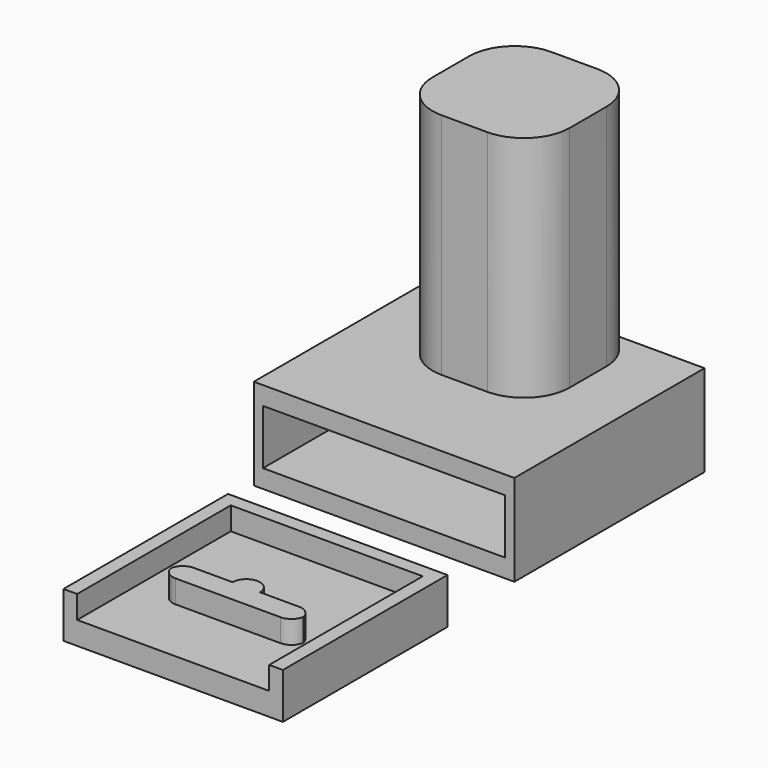
from build123d import *

# Parameters (mm, degrees)
F0_W        = 42
F0_H        = 39
F0_H_2      = 3
F1_DEPTH    = 5
F2_DEPTH    = 5
F3_T1_DEPTH = 12.5
F4_DEPTH    = 20
F0_W_2      = 53
F0_H_3      = 50
F5_DEPTH    = 4
F6_W        = 53
F6_H        = 4
F7_DEPTH    = 50
F8_W        = 30
F8_H        = 30
F9_DEPTH    = 50
F10_R       = 10


# Not quite as in the source:
# - a fillet or chamfer that OpenCascade refuses, or shapes differently, is made with other operations: its cross-section is extruded or revolved along the edge and cut away or added


with BuildPart() as f1:
    # F0 (on Top) → F1 (new body)
    with BuildSketch(Plane.XY):
        Rectangle(F0_W, F0_H)
        Polygon((-14.5, -7.5), (-14.5, -2.5), (-3, -2.5), (-3, 0.5), (3, 0.5), (3, -2.5), (14.5, -2.5), (14.5, -7.5), (3, -7.5), (-3, -7.5), align=None, mode=Mode.SUBTRACT)
        Polygon((-21, 19.5), (21, 19.5), (21, -19.5), (21, -22.5), (24, -22.5), (24, 22.5), (-24, 22.5), (-24, -22.5), (-21, -22.5), (-21, -19.5), align=None)
        with Locations((0, -21)):
            Rectangle(F0_W, F0_H_2)
        Polygon((-3, -2.5), (-14.5, -2.5), (-14.5, -7.5), (-3, -7.5), (3, -7.5), (14.5, -7.5), (14.5, -2.5), (3, -2.5), (3, 0.5), (-3, 0.5), align=None)
    extrude(amount=-F1_DEPTH)

    # F0 (on Top) → F2 (join)
    with BuildSketch(Plane.XY):
        Polygon((-3, -2.5), (-14.5, -2.5), (-14.5, -7.5), (-3, -7.5), (3, -7.5), (14.5, -7.5), (14.5, -2.5), (3, -2.5), (3, 0.5), (-3, 0.5), align=None)
        Polygon((-21, 19.5), (21, 19.5), (21, -19.5), (21, -22.5), (24, -22.5), (24, 22.5), (-24, 22.5), (-24, -22.5), (-21, -22.5), (-21, -19.5), align=None)
    extrude(amount=F2_DEPTH)

    # F3: fillet of radius 3 on 6 edges, made by hand

    # F3_s2 → F3_t1 (cut)
    with BuildSketch(Plane.XY):
        with BuildLine():
            ThreePointArc((-3, -2.5), (-2.1213203436, -0.3786796564), (0, 0.5))
            Line((0, 0.5), (-3, 0.5))
            Line((-3, 0.5), (-3, -2.5))
        make_face()
        with BuildLine():
            ThreePointArc((0, 0.5), (2.1213203436, -0.3786796564), (3, -2.5))
            Line((3, -2.5), (3, 0.5))
            Line((3, 0.5), (0, 0.5))
        make_face()
        with BuildLine():
            ThreePointArc((-14.5, -5.5), (-13.6213203436, -3.3786796564), (-11.5, -2.5))
            Line((-11.5, -2.5), (-14.5, -2.5))
            Line((-14.5, -2.5), (-14.5, -5.5))
        make_face()
        with BuildLine():
            ThreePointArc((-11.5, -7.5), (-13.6213203436, -6.6213203436), (-14.5, -4.5))
            Line((-14.5, -4.5), (-14.5, -7.5))
            Line((-14.5, -7.5), (-11.5, -7.5))
        make_face()
        with BuildLine():
            ThreePointArc((11.5, -2.5), (13.6213203436, -3.3786796564), (14.5, -5.5))
            Line((14.5, -5.5), (14.5, -2.5))
            Line((14.5, -2.5), (11.5, -2.5))
        make_face()
        with BuildLine():
            ThreePointArc((14.5, -4.5), (13.6213203436, -6.6213203436), (11.5, -7.5))
            Line((11.5, -7.5), (14.5, -7.5))
            Line((14.5, -7.5), (14.5, -4.5))
        make_face()
    extrude(amount=F3_T1_DEPTH, mode=Mode.SUBTRACT)


with BuildPart() as f4:
    # F0 (on Top) → F4 (new body)
    with BuildSketch(Plane.XY):
        Polygon((28.5, 35.1734315753), (28.5, 87.1734315753), (-28.5, 87.1734315753), (-28.5, 35.1734315753), (-26.5, 35.1734315753), (-26.5, 85.1734315753), (26.5, 85.1734315753), (26.5, 35.1734315753), align=None)
    extrude(amount=F4_DEPTH)

    # F0 (on Top) → F5 (join)
    with BuildSketch(Plane.XY):
        with Locations((0, 60.1734315753)):
            Rectangle(F0_W_2, F0_H_3)
    extrude(amount=F5_DEPTH)

    # F6 (on face) → F7 (join)
    with BuildSketch(Plane.XZ.offset(-85.1734315753)):
        with Locations((0, 18)):
            Rectangle(F6_W, F6_H)
    extrude(amount=F7_DEPTH)

    # F8 (on face) → F9 (join)
    with BuildSketch(Plane.XY.offset(20)):
        with Locations((0, 72.1734315753)):
            Rectangle(F8_W, F8_H)
    extrude(amount=F9_DEPTH)

    # F10
    f10_edges = [f4.edges().sort_by_distance(p)[0] for p in [
        (15, 57.173432, 45),
        (-15, 57.173432, 45),
        (-15, 87.173432, 45),
        (15, 87.173432, 45),
    ]]
    fillet(f10_edges, radius=F10_R)


solid = Compound([f1.part, f4.part])
